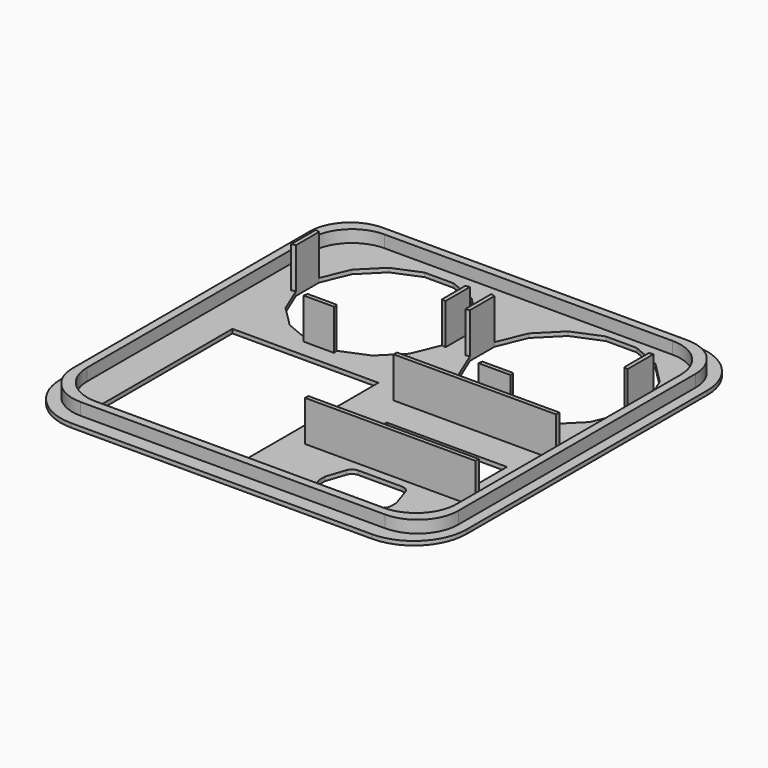
from build123d import *

# Parameters (mm, degrees)
F1_DEPTH  = 0.5
F4_DEPTH  = 1.5
F5_W      = 17.9758077912
F5_H      = 21.7117034923
F5_W_2    = 14.8
F5_H_2    = 6.5
F6_DEPTH  = 0.5
F7_W      = 21
F7_H      = 0.5
F8_DEPTH  = 5
F10_DEPTH = 5
F11_DEPTH = 0.5
F12_DEPTH = 0.5


# Not quite as in the source:
# - a feature names something its author has since deleted; it is built from what else it names


with BuildPart() as f1:
    # F0 (on Top) → F1 (new body)
    with BuildSketch(Plane.XY):
        with BuildLine():
            Line((43.5, 0), (6.5, 0))
            ThreePointArc((6.5, 0), (1.9038059223, -1.9038059223), (0, -6.5))
            Line((0, -6.5), (0, -43.5))
            ThreePointArc((0, -43.5), (1.9038059223, -48.0961940777), (6.5, -50))
            Line((6.5, -50), (43.5, -50))
            ThreePointArc((43.5, -50), (48.0961940777, -48.0961940777), (50, -43.5))
            Line((50, -43.5), (50, -6.5))
            ThreePointArc((50, -6.5), (48.0961940777, -1.9038059223), (43.5, 0))
        make_face()
    extrude(amount=F1_DEPTH)

    # F2 (on face) → F4 (join)
    with BuildSketch(Plane.XY.offset(0.5)):
        with BuildLine():
            Line((43.75, -1.75), (6.25, -1.75))
            ThreePointArc((6.25, -1.75), (2.7144660941, -3.2144660941), (1.25, -6.75))
            Line((1.25, -6.75), (1.25, -43.25))
            ThreePointArc((1.25, -43.25), (2.7144660941, -46.7855339059), (6.25, -48.25))
            Line((6.25, -48.25), (43.75, -48.25))
            ThreePointArc((43.75, -48.25), (47.2855339059, -46.7855339059), (48.75, -43.25))
            Line((48.75, -43.25), (48.75, -6.75))
            ThreePointArc((48.75, -6.75), (47.2855339059, -3.2144660941), (43.75, -1.75))
        make_face()
        with BuildLine():
            ThreePointArc((2.25, -7.75), (3.7144660941, -4.2144660941), (7.25, -2.75))
            Line((7.25, -2.75), (42.75, -2.75))
            ThreePointArc((42.75, -2.75), (46.2855339059, -4.2144660941), (47.75, -7.75))
            Line((47.75, -7.75), (47.75, -42.25))
            ThreePointArc((47.75, -42.25), (46.2855339059, -45.7855339059), (42.75, -47.25))
            Line((42.75, -47.25), (7.25, -47.25))
            ThreePointArc((7.25, -47.25), (3.7144660941, -45.7855339059), (2.25, -42.25))
            Line((2.25, -42.25), (2.25, -7.75))
        make_face(mode=Mode.SUBTRACT)
    extrude(amount=F4_DEPTH)

    # F5 (on face) → F6 (cut, through all)
    with BuildSketch(Plane(origin=(0, 0, 0), x_dir=(1, 0, 0), z_dir=(0, 0, -1))):
        with Locations((15.3125571672, 35.8414453501)):
            Rectangle(F5_W, F5_H)
        with BuildLine():
            Line((40.2913850072, 45.25), (33.4913850072, 45.25))
            ThreePointArc((33.4913850072, 45.25), (32.784278226, 44.9571067812), (32.4913850072, 44.25))
            Line((32.4913850072, 44.25), (32.4913850072, 43.45))
            Line((32.4913850072, 43.45), (33.2634609292, 41.133772234))
            ThreePointArc((33.2634609292, 41.133772234), (33.6274339426, 40.6387578148), (34.2121442272, 40.45))
            Line((34.2121442272, 40.45), (39.5706257871, 40.45))
            ThreePointArc((39.5706257871, 40.45), (40.1553360718, 40.6387578148), (40.5193090852, 41.133772234))
            Line((40.5193090852, 41.133772234), (41.2913850072, 43.45))
            Line((41.2913850072, 43.45), (41.2913850072, 44.25))
            ThreePointArc((41.2913850072, 44.25), (40.9984917884, 44.9571067812), (40.2913850072, 45.25))
        make_face()
        with Locations((37.5, 34.2)):
            Rectangle(F5_W_2, F5_H_2)
    extrude(amount=-F6_DEPTH, mode=Mode.SUBTRACT)

    # F7 (on face) → F8 (join)
    with BuildSketch(Plane.XY.offset(0.5)):
        with Locations((37.25, -39.1)):
            Rectangle(F7_W, F7_H)
        Polygon((37.75, -26.95), (47.75, -26.95), (47.75, -26.45), (27.75, -26.45), (27.75, -26.95), align=None)
    extrude(amount=F8_DEPTH)

    # F9 (on face) → F10 (join)
    with BuildSketch(Plane.XY.offset(0.5)):
        Polygon((46.7340297326, -11.4003978506), (46.7340297326, -15.1797328308), (47.2340297326, -15.2791890145), (47.2340297326, -11.3009416669), align=None)
        Polygon((39.1236972228, -22.7900653407), (35.3443622425, -22.7900653407), (35.2449060588, -23.2900653407), (39.2231534064, -23.2900653407), align=None)
        Polygon((27.2340297326, -15.2791890145), (27.7340297326, -15.1797328308), (27.7340297326, -11.4003978506), (27.2340297326, -11.3009416669), align=None)
        Polygon((17.1048343345, -22.7900653407), (17.0053781508, -22.2900653407), (13.424955538, -22.2900653407), (13.3254993543, -22.7900653407), align=None)
        Polygon((24.2151668444, -11.4998540343), (24.2151668444, -15.0802766471), (24.7151668444, -15.1797328308), (24.7151668444, -11.4003978506), align=None)
        Polygon((5.7151668444, -15.1797328308), (6.2151668444, -15.0802766471), (6.2151668444, -11.4998540343), (5.7151668444, -11.4003978506), align=None)
    extrude(amount=F10_DEPTH)

    # F9 (on face) → F11 (cut, through all)
    with BuildSketch(Plane.XY.offset(0.5)):
        Polygon((27.7340297326, -15.1797328308), (29.1803186149, -18.6713830655), (31.8527120078, -21.3437764584), (35.3443622425, -22.7900653407), (39.1236972228, -22.7900653407), (42.6153474575, -21.3437764584), (45.2877408504, -18.6713830655), (46.7340297326, -15.1797328308), (46.7340297326, -11.4003978506), (45.2877408504, -7.9087476159), (42.6153474575, -5.236354223), (39.1236972228, -3.7900653407), (35.3443622425, -3.7900653407), (31.8527120078, -5.236354223), (29.1803186149, -7.9087476159), (27.7340297326, -11.4003978506), align=None)
    extrude(amount=-F11_DEPTH, mode=Mode.SUBTRACT)

    # F9 (on face) → F12 (cut, through all)
    with BuildSketch(Plane.XY.offset(0.5)):
        Polygon((22.8449984296, -18.3881558169), (24.2151668444, -15.0802766471), (24.2151668444, -11.4998540343), (22.8449984296, -8.1919748645), (20.3132573206, -5.6602337555), (17.0053781508, -4.2900653407), (13.424955538, -4.2900653407), (10.1170763683, -5.6602337555), (7.5853352592, -8.1919748645), (6.2151668444, -11.4998540343), (6.2151668444, -15.0802766471), (7.5853352592, -18.3881558169), (10.1170763683, -20.9198969259), (13.424955538, -22.2900653407), (17.0053781508, -22.2900653407), (20.3132573206, -20.9198969259), align=None)
    extrude(amount=-F12_DEPTH, mode=Mode.SUBTRACT)


solid = f1.part
